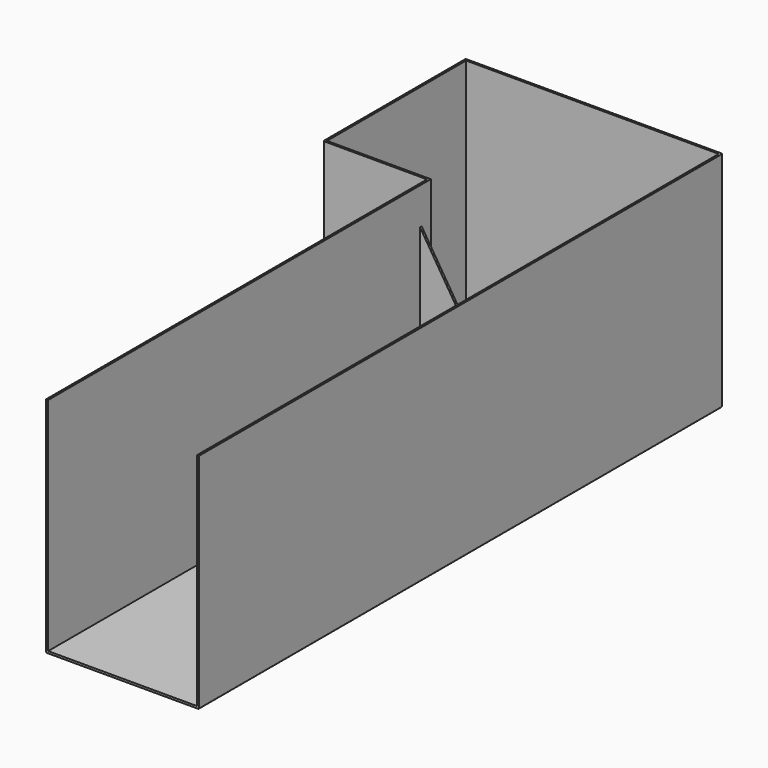
from build123d import *

# Parameters (mm, degrees)
F1_DEPTH  = 426
F3_DEPTH  = 4
F4_R      = 2
F7_DEPTH  = 4
F10_DEPTH = 4


# Not quite as in the source:
# - a feature names something its author has since deleted; it is built from what else it names


with BuildPart() as f1:
    # F0 (on Top) → F1 (new body)
    with BuildSketch(Plane.XY):
        Polygon((495, 0), (0, 0), (0, -343), (200, -343), (200, -1261), (204, -1261), (204, -339), (4, -339), (4, -4), (491, -4), (491, -1261), (495, -1261), align=None)
    extrude(amount=F1_DEPTH)

    # F2 (on Top) → F3 (join)
    with BuildSketch(Plane.XY):
        Polygon((0, -343), (200, -343), (200, -1261), (495, -1261), (495, 0), (0, 0), align=None)
    extrude(amount=-F3_DEPTH)

    # F4
    f4_edges = [f1.edges().sort_by_distance(p)[0] for p in [
        (100, -343, -4),
        (0, -171.5, -4),
        (247.5, 0, -4),
        (200, -343, 211),
        (0, -343, 211),
        (0, 0, 211),
        (495, 0, 211),
        (200, -802, -4),
        (495, -630.5, -4),
    ]]
    fillet(f4_edges, radius=F4_R)

    # F6 (on offset) → F7 (join)
    with BuildSketch(Plane.XZ.offset(961)):
        Polygon((269, 0), (491, 0), (491, 355), align=None)
    extrude(amount=F7_DEPTH)

    # F9 (on offset) → F10 (join)
    with BuildSketch(Plane.XZ.offset(361)):
        Polygon((204, 355), (204, 0), (426, 0), align=None)
    extrude(amount=F10_DEPTH)


solid = f1.part
